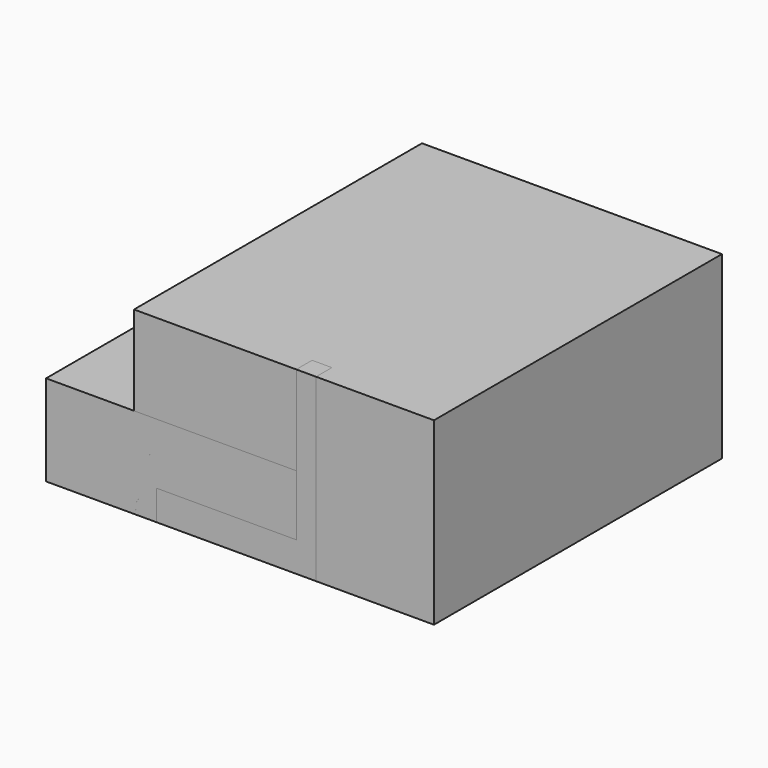
from build123d import *

# Parameters (mm, degrees)
F0_W   = 127
F0_H   = 152.4
F3_W   = 57.15
F3_H   = 20.3735902905
F3_H_2 = 23.6665979028
F3_H_3 = 22.5742906332
F6_W   = 67.564
F6_H   = 47.498
F9_W   = 8.382
F9_H   = 63.5


with BuildPart() as f2:
    # F2: sweep along a path in F1
    with BuildLine(Plane.YZ) as f2_path:
        Line((0, 0), (0, 76.2))
    # F0 (on Top) → F2 (sweep)
    with BuildSketch(Plane.XY):
        with Locations((-13.5811662078, 76.2)):
            Rectangle(F0_W, F0_H)
    sweep(path=f2_path.line)


with BuildPart() as f5:
    # F5: sweep along a path in F4
    with BuildLine(Plane.YZ) as f5_path:
        Line((0, 0), (0, 38.4406633675))
    # F3 (on Top) → F5 (sweep)
    with BuildSketch(Plane.XY):
        with Locations((-28.575, 10.1867951453)):
            Rectangle(F3_W, F3_H)
        with Locations((-85.725, 10.1867951453)):
            Rectangle(F3_W, F3_H)
        with Locations((-85.725, 32.2068892419)):
            Rectangle(F3_W, F3_H_2)
        with Locations((-28.575, 32.2068892419)):
            Rectangle(F3_W, F3_H_2)
        with Locations((-28.575, 55.3273335099)):
            Rectangle(F3_W, F3_H_3)
        with Locations((-85.725, 55.3273335099)):
            Rectangle(F3_W, F3_H_3)
    sweep(path=f5_path.line)


with BuildPart() as f8:
    # F8: sweep along a path in F7
    with BuildLine(Plane.YZ) as f8_path:
        Line((0, 0), (0, 12.7))
    # F6 (on Top) → F8 (sweep)
    with BuildSketch(Plane.XY):
        with Locations((-33.782, 23.749)):
            Rectangle(F6_W, F6_H)
    sweep(path=f8_path.line)

    # F11: sweep along a path in F10
    with BuildLine(Plane.XZ) as f11_path:
        Line((0, 12.7), (-8.382, 12.7))
    # F9 (on Right) → F11 (sweep)
    with BuildSketch(Plane.YZ):
        with Locations((4.191, 44.45)):
            Rectangle(F9_W, F9_H)
    sweep(path=f11_path.line)


solid = Compound([f2.part, f5.part, f8.part])
